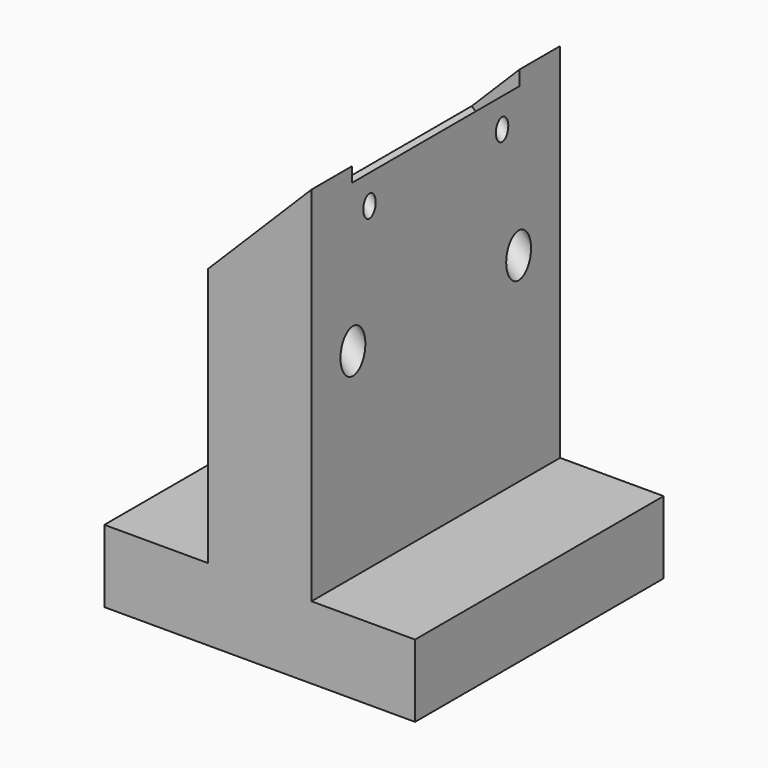
from build123d import *

# Parameters (mm, degrees)
F0_W        = 30
F0_H        = 30
F1_DEPTH    = 7
F2_W        = 10
F2_H        = 30
F3_DEPTH    = 35
F4_T1_DEPTH = 81.4336597593
F5_W        = 25.2
F5_H        = 25.2
F6_DEPTH    = 2
F9_D        = 2.5
F9_DEPTH    = 16.5
F9_TIP      = 0.7510757738
F10_W       = 20.2
F10_H       = 6.5
F11_DEPTH   = 1
F14_D       = 1.5
F16_D       = 3


# Not quite as in the source:
# - a fillet or chamfer that OpenCascade refuses, or shapes differently, is made with other operations: its cross-section is extruded or revolved along the edge and cut away or added


with BuildPart() as f1:
    # F0 (on Top) → F1 (new body)
    with BuildSketch(Plane.XY):
        Rectangle(F0_W, F0_H)
    extrude(amount=F1_DEPTH)

    # F2 (on face) → F3 (join)
    with BuildSketch(Plane.XY.offset(7)):
        Rectangle(F2_W, F2_H)
    extrude(amount=F3_DEPTH)

    # F4: chamfer of 10 on 1 edges, made by hand

    # F4_s2 → F4_t1 (cut)
    with BuildSketch(Plane.XZ.offset(-40.7168298797)):
        Polygon((-5, 32), (5, 42), (-5, 42), align=None)
    extrude(amount=F4_T1_DEPTH, mode=Mode.SUBTRACT)


with BuildPart() as f6:
    # F5 (on face) → F6 (new body)
    with BuildSketch(Plane(origin=(0, 0, 0), x_dir=(1, 0, 0), z_dir=(0, 0, -1))):
        Rectangle(F5_W, F5_H)
    extrude(amount=-F6_DEPTH)


with BuildPart() as f1_1:
    add(f1.part)

    # F7: cut F6
    add(f6.part, mode=Mode.SUBTRACT)

    # F9
    with Locations(Plane(origin=(0, 0, 2), x_dir=(1, 0, 0), z_dir=(0, 0, -1))):
        with Locations((0, 0)):
            Hole(F9_D / 2, depth=F9_DEPTH)
            with Locations((0, 0, -(F9_DEPTH + F9_TIP / 2))):  # 118° drill point
                Cone(0, F9_D / 2, F9_TIP, mode=Mode.SUBTRACT)


with BuildPart() as f11:
    # F10 (on face) → F11 (new body)
    with BuildSketch(Plane(origin=(-18.5, 0, 18.5), x_dir=(0, -1, 0), z_dir=(-0.7071067812, 0, 0.7071067812))):
        with Locations((0, 29.9840187158)):
            Rectangle(F10_W, F10_H)
    extrude(amount=-F11_DEPTH)


with BuildPart() as f1_2:
    add(f1_1.part)

    # F12: cut F11
    add(f11.part, mode=Mode.SUBTRACT)

    # F14 (through all)
    with Locations(Plane(origin=(-17.7928932188, 0, 17.7928932188), x_dir=(0, -1, 0), z_dir=(-0.7071067812, 0, 0.7071067812))):
        with Locations((-8, 30.2340187158), (8, 30.2340187158)):
            Hole(F14_D / 2)

    # F16 (through all)
    with Locations(Plane(origin=(-18.5, 0, 18.5), x_dir=(0, -1, 0), z_dir=(-0.7071067812, 0, 0.7071067812))):
        with Locations((-10, 22.091883092), (10, 22.091883092)):
            Hole(F16_D / 2)


solid = f1_2.part
